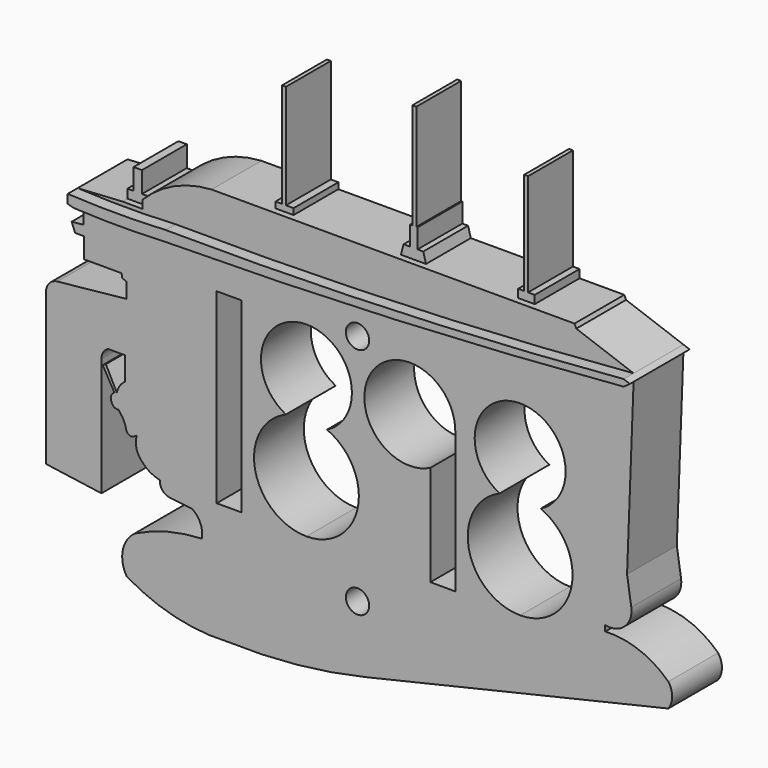
from build123d import *

# Parameters (mm, degrees)
F1_DEPTH = 12.7
F2_DEPTH = 12.7
F3_DEPTH = 15.24
F0_W     = 0.8031209019
F0_H     = 20.8792375506
F0_H_2   = 21.3003987877
F0_H_3   = 21.5899625402
F4_DEPTH = 11.43
F6_W     = 5.08
F6_H     = 38.1
F6_R     = 4.1999289977
F7_DEPTH = 25.4
F9_DEPTH = 25.4


# Not quite as in the source:
# - a feature names something its author has since deleted; it is built from what else it names


with BuildPart() as f1:
    # F0 (on Front) → F1 (new body)
    with BuildSketch(Plane.XZ):
        with BuildLine():
            Line((-48.7551556499, 16.502033492), (-48.7551556499, 13.4174126565))
            Line((-48.7551556499, 13.4174126565), (-62.8553717881, 11.9587710013))
            ThreePointArc((-62.8553717881, 11.9587710013), (-64.4593193904, 11.1699658138), (-65.1648855989, 9.527699739))
            Line((-65.1648855989, 9.527699739), (-65.1648855989, -21.5900078871))
            Line((-65.1648855989, -21.5900078871), (-53.8604057294, -23.1702051567))
            Line((-53.8604057294, -23.1702051567), (-53.8604057294, 1.0189516987))
            ThreePointArc((-53.8604057294, 1.0189516987), (-53.4996704115, 2.3010390091), (-52.5233172394, 3.2069155593))
            Line((-52.5233172394, 3.2069155593), (-49.036793639, 3.2069155593))
            Line((-49.036793639, 3.2069155593), (-49.036793639, -1.5386344666))
            ThreePointArc((-49.036793639, -1.5386344666), (-47.615617645, -3.4104534246), (-47.3704157715, -5.7478287601))
            Line((-47.3704157715, -5.7478287601), (-46.9190361118, -6.2988243644))
            ThreePointArc((-46.9190361118, -6.2988243644), (-46.2448724821, -6.7832935586), (-45.6504018941, -7.3627861985))
            ThreePointArc((-45.6504018941, -7.3627861985), (-45.2851101067, -8.4586657322), (-45.6504018941, -9.5545452658))
            ThreePointArc((-45.6504018941, -9.5545452658), (-46.1279766102, -10.0258883196), (-46.6583830297, -10.4368760494))
            ThreePointArc((-46.6583830297, -10.4368760494), (-46.8361198696, -11.8225114542), (-46.60965919, -13.2010220344))
            ThreePointArc((-46.60965919, -13.2010220344), (-44.7140636791, -15.6159662106), (-41.9303173119, -16.9105680327))
            ThreePointArc((-41.9303173119, -16.9105680327), (-41.4025572934, -18.5951701498), (-39.849619977, -19.4346941943))
            Line((-39.849619977, -19.4346941943), (-35.3891622198, -19.9264425199))
            ThreePointArc((-35.3891622198, -19.9264425199), (-25.5608590414, -18.8572797934), (-15.7824102789, -17.4010545015))
            ThreePointArc((-15.7824102789, -17.4010545015), (-8.2182486661, -13.3883283665), (-5.1937012606, -5.3776714064))
            Line((-5.1937012606, -5.3776714064), (38.9031486872, 1.6952896796))
            Line((38.9031486872, 1.6952896796), (48.6844740711, 1.6952896796))
            Line((48.6844740711, 1.6952896796), (48.9549487829, -13.394898735))
            ThreePointArc((48.9549487829, -13.394898735), (52.9202633868, -12.3483898503), (54.2744512358, -8.4773336607))
            Line((54.2744512358, -8.4773336607), (53.4126908814, -2.8367075716))
            Line((53.4126908814, -2.8367075716), (54.7520132328, 32.3448944531))
            ThreePointArc((54.7520132328, 32.3448944531), (8.06619556, 29.2264265692), (-38.7060455978, 27.9427323651))
            ThreePointArc((-38.7060455978, 27.9427323651), (-48.0915364769, 27.7060167093), (-57.477027356, 27.9427323651))
            Line((-57.477027356, 27.9427323651), (-57.477027356, 23.904802117))
            Line((-57.477027356, 23.904802117), (-59.946908801, 23.649297384))
            Line((-59.946908801, 23.649297384), (-59.2430122304, 21.8624826357))
            Line((-59.2430122304, 21.8624826357), (-57.4561974821, 21.8624826357))
            Line((-57.4561974821, 21.8624826357), (-57.4561974821, 17.7166229842))
            Line((-57.4561974821, 17.7166229842), (-49.7400154939, 17.7166229842))
            Line((-49.7400154939, 17.7166229842), (-49.6591787643, 16.9352005181))
            Line((-49.6591787643, 16.9352005181), (-48.7551556499, 16.502033492))
        make_face()
        with BuildLine():
            ThreePointArc((-47.3704157715, -5.7478287601), (-47.615617645, -3.4104534246), (-49.036793639, -1.5386344666))
            ThreePointArc((-49.036793639, -1.5386344666), (-50.1207303597, -2.6383216139), (-50.7394958839, -4.0530158787))
            ThreePointArc((-50.7394958839, -4.0530158787), (-49.7106058857, -4.489200491), (-49.2601067453, -5.5119038542))
            ThreePointArc((-49.2601067453, -5.5119038542), (-48.3211852646, -5.6888381711), (-47.4264473374, -6.0239849165))
            ThreePointArc((-47.4264473374, -6.0239849165), (-47.3962036519, -5.8863588755), (-47.3704157715, -5.7478287601))
        make_face()
        with BuildLine():
            ThreePointArc((-49.2601067453, -5.5119038542), (-49.7106058857, -4.489200491), (-50.7394958839, -4.0530158787))
            ThreePointArc((-50.7394958839, -4.0530158787), (-50.8140907016, -5.5738489648), (-50.3470855905, -7.0231259877))
            ThreePointArc((-50.3470855905, -7.0231259877), (-49.5443514855, -6.4539822041), (-49.2601067453, -5.5119038542))
        make_face()
        with BuildLine():
            ThreePointArc((-50.3470855905, -7.0231259877), (-50.8140907016, -5.5738489648), (-50.7394958839, -4.0530158787))
            ThreePointArc((-50.7394958839, -4.0530158787), (-50.9812103214, -4.1166962613), (-51.2089185655, -4.2197982303))
            ThreePointArc((-51.2089185655, -4.2197982303), (-51.743532248, -4.7258542326), (-51.9714604077, -5.4258208183))
            ThreePointArc((-51.9714604077, -5.4258208183), (-51.7264168334, -6.2602547319), (-51.186346321, -6.9419072469))
            ThreePointArc((-51.186346321, -6.9419072469), (-50.7704583506, -7.0211880502), (-50.3470855905, -7.0231259877))
        make_face()
        with BuildLine():
            ThreePointArc((-51.2089185655, -4.2197982303), (-50.9812103214, -4.1166962613), (-50.7394958839, -4.0530158787))
            Line((-50.7394958839, -4.0530158787), (-52.958683025, 0.3205834158))
            Line((-52.958683025, 0.3205834158), (-53.6059290171, -0.051631916))
            Line((-53.6059290171, -0.051631916), (-51.2089185655, -4.2197982303))
        make_face()
        with BuildLine():
            Line((-46.9190361118, -6.2988243644), (-47.3704157715, -5.7478287601))
            ThreePointArc((-47.3704157715, -5.7478287601), (-47.3962036519, -5.8863588755), (-47.4264473374, -6.0239849165))
            ThreePointArc((-47.4264473374, -6.0239849165), (-47.1691719509, -6.15481409), (-46.9190361118, -6.2988243644))
        make_face()
        with BuildLine():
            ThreePointArc((-49.5964513737, -8.0300319781), (-49.946242615, -7.507549809), (-50.3470855905, -7.0231259877))
            ThreePointArc((-50.3470855905, -7.0231259877), (-50.0092212706, -7.5544995086), (-49.5964513737, -8.0300319781))
        make_face()
        with BuildLine():
            ThreePointArc((-49.2601067453, -5.5119038542), (-49.5443514855, -6.4539822041), (-50.3470855905, -7.0231259877))
            ThreePointArc((-50.3470855905, -7.0231259877), (-49.946242615, -7.507549809), (-49.5964513737, -8.0300319781))
            ThreePointArc((-49.5964513737, -8.0300319781), (-49.3266753815, -8.2757089525), (-49.036793639, -8.4973050651))
            ThreePointArc((-49.036793639, -8.4973050651), (-48.0163521737, -7.4008033663), (-47.4264473374, -6.0239849165))
            ThreePointArc((-47.4264473374, -6.0239849165), (-48.3211852646, -5.6888381711), (-49.2601067453, -5.5119038542))
        make_face()
        with BuildLine():
            ThreePointArc((-46.9190361118, -6.2988243644), (-47.1691719509, -6.15481409), (-47.4264473374, -6.0239849165))
            ThreePointArc((-47.4264473374, -6.0239849165), (-48.0163521737, -7.4008033663), (-49.036793639, -8.4973050651))
            ThreePointArc((-49.036793639, -8.4973050651), (-49.3266753815, -8.2757089525), (-49.5964513737, -8.0300319781))
            ThreePointArc((-49.5964513737, -8.0300319781), (-49.1268650573, -8.9954240946), (-48.8306023576, -10.0272776016))
            ThreePointArc((-48.8306023576, -10.0272776016), (-48.4443790706, -10.7265299049), (-47.6917445685, -10.9942303294))
            ThreePointArc((-47.6917445685, -10.9942303294), (-47.1604512125, -10.7426456251), (-46.6583830297, -10.4368760494))
            ThreePointArc((-46.6583830297, -10.4368760494), (-46.6347395299, -10.3551418199), (-46.60965919, -10.2738369867))
            ThreePointArc((-46.60965919, -10.2738369867), (-45.8234576817, -8.6803013071), (-46.356693987, -6.9852709782))
            Line((-46.356693987, -6.9852709782), (-46.9190361118, -6.2988243644))
        make_face()
        with BuildLine():
            ThreePointArc((-45.6504018941, -7.3627861985), (-46.2448724821, -6.7832935586), (-46.9190361118, -6.2988243644))
            Line((-46.9190361118, -6.2988243644), (-46.356693987, -6.9852709782))
            ThreePointArc((-46.356693987, -6.9852709782), (-45.8234576817, -8.6803013071), (-46.60965919, -10.2738369867))
            ThreePointArc((-46.60965919, -10.2738369867), (-46.6347395299, -10.3551418199), (-46.6583830297, -10.4368760494))
            ThreePointArc((-46.6583830297, -10.4368760494), (-46.1279766102, -10.0258883196), (-45.6504018941, -9.5545452658))
            ThreePointArc((-45.6504018941, -9.5545452658), (-45.2851101067, -8.4586657322), (-45.6504018941, -7.3627861985))
        make_face()
        Polygon((48.9549487829, -14.5681889131), (48.9549487829, -13.394898735), (48.6844740711, 1.6952896796), (0, -6.1135082506), (0, -33.2036390901), (6.9897733629, -31.6629558802), (6.9897733629, -12.1476817876), (44.0394468606, -6.2050600536), (44.0394468606, -23.5927309841), (48.9549487829, -22.5092579032), align=None)
        with BuildLine():
            ThreePointArc((61.8351144011, -19.3772837126), (55.8950908573, -15.6334310122), (48.9549487829, -14.5681889131))
            Line((48.9549487829, -14.5681889131), (48.9549487829, -22.5092579032))
            Line((48.9549487829, -22.5092579032), (44.0394468606, -23.5927309841))
            Line((44.0394468606, -23.5927309841), (6.9897733629, -31.6629558802))
            Line((6.9897733629, -31.6629558802), (0, -33.2036390901))
            ThreePointArc((0, -33.2036390901), (-13.9786608203, -35.5041994352), (-28.1235985458, -36.2892299891))
            ThreePointArc((-28.1235985458, -36.2892299891), (-36.968923327, -35.9627176522), (-45.3792661428, -33.2036390901))
            ThreePointArc((-45.3792661428, -33.2036390901), (-46.9884285215, -30.9374841749), (-47.0181743808, -28.1582798204))
            ThreePointArc((-47.0181743808, -28.1582798204), (-49.5076846975, -31.9569932635), (-48.7172485904, -36.4294753708))
            ThreePointArc((-48.7172485904, -36.4294753708), (-38.8219806126, -40.4819745273), (-28.1747894096, -41.4701026827))
            ThreePointArc((-28.1747894096, -41.4701026827), (-13.9958743449, -40.9971425936), (0, -38.6774820627))
            Line((0, -38.6774820627), (61.8351144011, -24.218985916))
            ThreePointArc((61.8351144011, -24.218985916), (62.6222056643, -21.7981348143), (61.8351144011, -19.3772837126))
        make_face()
        Polygon((0, -6.1135082506), (48.6844740711, 1.6952896796), (38.9031486872, 1.6952896796), (-5.1937012606, -5.3776714064), align=None)
        Polygon((0, -33.2036390901), (0, -6.1135082506), (-5.1937012606, -5.3776714064), (-5.1937012606, -31.4487681253), align=None)
        with BuildLine():
            ThreePointArc((-15.7824102789, -17.4010545015), (-25.5608590414, -18.8572797934), (-35.3891622198, -19.9264425199))
            ThreePointArc((-35.3891622198, -19.9264425199), (-33.6624013857, -21.9793164564), (-33.3946987915, -24.6484604575))
            Line((-33.3946987915, -24.6484604575), (-33.3946987915, -29.0951598436))
            Line((-33.3946987915, -29.0951598436), (-28.4458585083, -27.9946736991))
            Line((-28.4458585083, -27.9946736991), (-28.4458585083, -31.1493985355))
            Line((-28.4458585083, -31.1493985355), (-16.4138842374, -28.6549646407))
            Line((-16.4138842374, -28.6549646407), (-17.5877343863, -27.2610168904))
            Line((-17.5877343863, -27.2610168904), (-5.1937012606, -31.4487681253))
            Line((-5.1937012606, -31.4487681253), (-5.1937012606, -5.3776714064))
            ThreePointArc((-5.1937012606, -5.3776714064), (-8.2182486661, -13.3883283665), (-15.7824102789, -17.4010545015))
        make_face()
        Polygon((6.9897733629, -31.6629558802), (44.0394468606, -23.5927309841), (44.0394468606, -6.2050600536), (6.9897733629, -12.1476817876), align=None)
        with BuildLine():
            ThreePointArc((-28.1235985458, -36.2892299891), (-13.9786608203, -35.5041994352), (0, -33.2036390901))
            Line((0, -33.2036390901), (-5.1937012606, -31.4487681253))
            Line((-5.1937012606, -31.4487681253), (-17.5877343863, -27.2610168904))
            Line((-17.5877343863, -27.2610168904), (-16.4138842374, -28.6549646407))
            Line((-16.4138842374, -28.6549646407), (-28.4458585083, -31.1493985355))
            Line((-28.4458585083, -31.1493985355), (-28.4458585083, -27.9946736991))
            Line((-28.4458585083, -27.9946736991), (-33.3946987915, -29.0951598436))
            Line((-33.3946987915, -29.0951598436), (-33.3946987915, -24.6484604575))
            ThreePointArc((-33.3946987915, -24.6484604575), (-40.3900375793, -25.6907170392), (-47.0181743808, -28.1582798204))
            ThreePointArc((-47.0181743808, -28.1582798204), (-46.9884285215, -30.9374841749), (-45.3792661428, -33.2036390901))
            ThreePointArc((-45.3792661428, -33.2036390901), (-36.968923327, -35.9627176522), (-28.1235985458, -36.2892299891))
        make_face()
    extrude(amount=F1_DEPTH)



with BuildPart() as f1b:
    # F0 (on Front) → F1, piece 2 (new body)
    with BuildSketch(Plane.XZ):
        with BuildLine():
            Line((-49.5634950364, 30.6502017175), (-58.7173150909, 30.0915159325))
            ThreePointArc((-58.7173150909, 30.0915159325), (-48.7116803443, 29.8224606957), (-38.7060455978, 30.0915159325))
            ThreePointArc((-38.7060455978, 30.0915159325), (8.0657939775, 30.8005791155), (54.7520132328, 33.7168574792))
            Line((54.7520132328, 33.7168574792), (43.0524877201, 37.9363596424))
            Line((43.0524877201, 37.9363596424), (42.6878245507, 38.7264558278))
            Line((42.6878245507, 38.7264558278), (33.556767168, 38.7264558278))
            Line((33.556767168, 38.7264558278), (30.1818160021, 38.7264558278))
            Line((30.1818160021, 38.7264558278), (11.3595948708, 38.7264558278))
            Line((11.3595948708, 38.7264558278), (6.237627371, 38.7264558278))
            Line((6.237627371, 38.7264558278), (-15.6707727532, 38.7264558278))
            Line((-15.6707727532, 38.7264558278), (-19.3496172971, 38.7264558278))
            Line((-19.3496172971, 38.7264558278), (-31.3758637064, 38.7264558278))
            ThreePointArc((-31.3758637064, 38.7264558278), (-39.0221039671, 36.8382050442), (-45.4714367213, 32.3175205636))
            Line((-45.4714367213, 32.3175205636), (-45.4714367213, 30.6502017175))
            Line((-45.4714367213, 30.6502017175), (-49.5634950364, 30.6502017175))
        make_face()
    extrude(amount=F1_DEPTH)


with BuildPart() as f2:
    # F0 (on Front) → F2 (new body)
    with BuildSketch(Plane.XZ):
        with BuildLine():
            ThreePointArc((-46.9190361118, -6.2988243644), (-47.1691719509, -6.15481409), (-47.4264473374, -6.0239849165))
            ThreePointArc((-47.4264473374, -6.0239849165), (-48.0163521737, -7.4008033663), (-49.036793639, -8.4973050651))
            ThreePointArc((-49.036793639, -8.4973050651), (-49.3266753815, -8.2757089525), (-49.5964513737, -8.0300319781))
            ThreePointArc((-49.5964513737, -8.0300319781), (-49.1268650573, -8.9954240946), (-48.8306023576, -10.0272776016))
            ThreePointArc((-48.8306023576, -10.0272776016), (-48.4443790706, -10.7265299049), (-47.6917445685, -10.9942303294))
            ThreePointArc((-47.6917445685, -10.9942303294), (-47.1604512125, -10.7426456251), (-46.6583830297, -10.4368760494))
            ThreePointArc((-46.6583830297, -10.4368760494), (-46.6347395299, -10.3551418199), (-46.60965919, -10.2738369867))
            ThreePointArc((-46.60965919, -10.2738369867), (-45.8234576817, -8.6803013071), (-46.356693987, -6.9852709782))
            Line((-46.356693987, -6.9852709782), (-46.9190361118, -6.2988243644))
        make_face()
        with BuildLine():
            ThreePointArc((-49.2601067453, -5.5119038542), (-49.5443514855, -6.4539822041), (-50.3470855905, -7.0231259877))
            ThreePointArc((-50.3470855905, -7.0231259877), (-49.946242615, -7.507549809), (-49.5964513737, -8.0300319781))
            ThreePointArc((-49.5964513737, -8.0300319781), (-49.3266753815, -8.2757089525), (-49.036793639, -8.4973050651))
            ThreePointArc((-49.036793639, -8.4973050651), (-48.0163521737, -7.4008033663), (-47.4264473374, -6.0239849165))
            ThreePointArc((-47.4264473374, -6.0239849165), (-48.3211852646, -5.6888381711), (-49.2601067453, -5.5119038542))
        make_face()
        with BuildLine():
            ThreePointArc((-45.6504018941, -7.3627861985), (-46.2448724821, -6.7832935586), (-46.9190361118, -6.2988243644))
            Line((-46.9190361118, -6.2988243644), (-46.356693987, -6.9852709782))
            ThreePointArc((-46.356693987, -6.9852709782), (-45.8234576817, -8.6803013071), (-46.60965919, -10.2738369867))
            ThreePointArc((-46.60965919, -10.2738369867), (-46.6347395299, -10.3551418199), (-46.6583830297, -10.4368760494))
            ThreePointArc((-46.6583830297, -10.4368760494), (-46.1279766102, -10.0258883196), (-45.6504018941, -9.5545452658))
            ThreePointArc((-45.6504018941, -9.5545452658), (-45.2851101067, -8.4586657322), (-45.6504018941, -7.3627861985))
        make_face()
        with BuildLine():
            Line((-46.9190361118, -6.2988243644), (-47.3704157715, -5.7478287601))
            ThreePointArc((-47.3704157715, -5.7478287601), (-47.3962036519, -5.8863588755), (-47.4264473374, -6.0239849165))
            ThreePointArc((-47.4264473374, -6.0239849165), (-47.1691719509, -6.15481409), (-46.9190361118, -6.2988243644))
        make_face()
        with BuildLine():
            ThreePointArc((-49.2601067453, -5.5119038542), (-49.7106058857, -4.489200491), (-50.7394958839, -4.0530158787))
            ThreePointArc((-50.7394958839, -4.0530158787), (-50.8140907016, -5.5738489648), (-50.3470855905, -7.0231259877))
            ThreePointArc((-50.3470855905, -7.0231259877), (-49.5443514855, -6.4539822041), (-49.2601067453, -5.5119038542))
        make_face()
    extrude(amount=F2_DEPTH)


with BuildPart() as f1_1:
    add(f1.part)

    add(f1b.part)  # F3 merges F1b
    # F0 (on Front) → F3 (join)
    with BuildSketch(Plane.XZ):
        with BuildLine():
            Line((-58.7173150909, 28.2865388137), (-57.477027356, 27.9427323651))
            ThreePointArc((-57.477027356, 27.9427323651), (-48.0915364769, 27.7060167093), (-38.7060455978, 27.9427323651))
            ThreePointArc((-38.7060455978, 27.9427323651), (8.06619556, 29.2264265692), (54.7520132328, 32.3448944531))
            Line((54.7520132328, 32.3448944531), (56.0283269774, 33.2565474777))
            Line((56.0283269774, 33.2565474777), (54.7520132328, 33.7168574792))
            ThreePointArc((54.7520132328, 33.7168574792), (8.0657939775, 30.8005791155), (-38.7060455978, 30.0915159325))
            ThreePointArc((-38.7060455978, 30.0915159325), (-48.7116803443, 29.8224606957), (-58.7173150909, 30.0915159325))
            Line((-58.7173150909, 30.0915159325), (-58.7173150909, 28.2865388137))
        make_face()
    extrude(amount=F3_DEPTH)

    # F0 (on Front) → F4 (join)
    with BuildSketch(Plane.XZ):
        Polygon((-49.5634950364, 32.4551788364), (-49.5634950364, 30.6502017175), (-45.4714367213, 30.6502017175), (-45.4714367213, 32.3175205636), (-45.4714367213, 32.4551788364), (-46.6116432115, 32.4551788364), (-46.6116432115, 36.7413145776), (-48.3172012532, 36.7413145776), (-48.3172012532, 32.4551788364), align=None)
        Polygon((-19.3496172971, 39.9737632714), (-19.3496172971, 38.7264558278), (-15.6707727532, 38.7264558278), (-15.6707727532, 39.9737632714), (-17.2171857255, 39.9737632714), (-18.0203066274, 39.9737632714), align=None)
        Polygon((6.7892512256, 40.7851440797), (6.237627371, 38.7264558278), (11.3595948708, 38.7264558278), (10.8079710163, 40.7851440797), (9.6353090061, 40.7851440797), (9.6353090061, 44.7442179937), (9.3757620237, 44.7442179937), (8.5726411218, 44.7442179937), (8.1109651281, 44.7442179937), (8.1109651281, 40.7851440797), align=None)
        with Locations((31.7935269116, 50.8345432838)):
            Rectangle(F0_W, F0_H)
        Polygon((30.1818160021, 38.7264558278), (33.556767168, 38.7264558278), (33.556767168, 40.3949245085), (32.1950873626, 40.3949245085), (31.3919664607, 40.3949245085), (30.1818160021, 40.3949245085), align=None)
        with Locations((-17.6187461764, 50.6239626653)):
            Rectangle(F0_W, F0_H_2)
        with Locations((8.9742015728, 55.5391992638)):
            Rectangle(F0_W, F0_H_3)
    extrude(amount=F4_DEPTH)


with BuildPart() as f2_1:
    add(f2.part)

    # F5: union F1
    add(f1_1.part)

    # F6 (on face) → F7 (cut)
    with BuildSketch(Plane.XZ.offset(12.7)):
        with Locations((-27.8038021288, 1.7426949936)):
            Rectangle(F6_W, F6_H)
        with BuildLine():
            Line((-12.0248878375, 16.1970947476), (-12.0248878375, 20.7926949936))
            ThreePointArc((-12.0248878375, 20.7926949936), (-21.0509501852, 13.6685212457), (-16.2184503735, 3.2344137772))
            ThreePointArc((-16.2184503735, 3.2344137772), (-14.1649165015, 3.8743114334), (-12.0248878375, 4.0905235764))
            Line((-12.0248878375, 4.0905235764), (-12.0248878375, 6.8284372443))
            ThreePointArc((-12.0248878375, 6.8284372443), (-16.7092165891, 11.512765996), (-12.0248878375, 16.1970947476))
        make_face()
        with BuildLine():
            ThreePointArc((-2.7449588398, 11.512765996), (-5.4629871143, 18.0746667192), (-12.0248878375, 20.7926949936))
            Line((-12.0248878375, 20.7926949936), (-12.0248878375, 16.1970947476))
            ThreePointArc((-12.0248878375, 16.1970947476), (-8.7125672119, 14.8250866216), (-7.3405590858, 11.512765996))
            ThreePointArc((-7.3405590858, 11.512765996), (-8.7125672119, 8.2004453704), (-12.0248878375, 6.8284372443))
            Line((-12.0248878375, 6.8284372443), (-12.0248878375, 4.0905235764))
            ThreePointArc((-12.0248878375, 4.0905235764), (-9.8848591734, 3.8743114334), (-7.8313253015, 3.2344137772))
            ThreePointArc((-7.8313253015, 3.2344137772), (-4.1181487883, 6.6547252582), (-2.7449588398, 11.512765996))
        make_face()
        with BuildLine():
            ThreePointArc((-12.0248878375, 2.2328369983), (-9.8691325877, 2.4867036483), (-7.8313253015, 3.2344137772))
            ThreePointArc((-7.8313253015, 3.2344137772), (-9.8848591734, 3.8743114334), (-12.0248878375, 4.0905235764))
            Line((-12.0248878375, 4.0905235764), (-12.0248878375, 2.2328369983))
        make_face()
        with BuildLine():
            ThreePointArc((-12.0248878375, 4.0905235764), (-14.1649165015, 3.8743114334), (-16.2184503735, 3.2344137772))
            ThreePointArc((-16.2184503735, 3.2344137772), (-14.1806430872, 2.4867036483), (-12.0248878375, 2.2328369983))
            Line((-12.0248878375, 2.2328369983), (-12.0248878375, 4.0905235764))
        make_face()
        with BuildLine():
            ThreePointArc((-16.2184503735, 3.2344137772), (-22.5075899858, -8.748419379), (-12.0248878375, -17.3073050064))
            Line((-12.0248878375, -17.3073050064), (-12.0248878375, -12.3384351215))
            ThreePointArc((-12.0248878375, -12.3384351215), (-17.754932244, -6.608390715), (-12.0248878375, -0.8783463084))
            Line((-12.0248878375, -0.8783463084), (-12.0248878375, 2.2328369983))
            ThreePointArc((-12.0248878375, 2.2328369983), (-14.1806430872, 2.4867036483), (-16.2184503735, 3.2344137772))
        make_face()
        with BuildLine():
            Line((-12.0248878375, -12.3384351215), (-12.0248878375, -17.3073050064))
            ThreePointArc((-12.0248878375, -17.3073050064), (-4.4596129907, -14.1736655617), (-1.3259735461, -6.608390715))
            ThreePointArc((-1.3259735461, -6.608390715), (-3.0992692829, -0.709229721), (-7.8313253015, 3.2344137772))
            ThreePointArc((-7.8313253015, 3.2344137772), (-9.8691325877, 2.4867036483), (-12.0248878375, 2.2328369983))
            Line((-12.0248878375, 2.2328369983), (-12.0248878375, -0.8783463084))
            ThreePointArc((-12.0248878375, -0.8783463084), (-7.9731345811, -2.5566374586), (-6.2948434309, -6.608390715))
            ThreePointArc((-6.2948434309, -6.608390715), (-7.9731345811, -10.6601439714), (-12.0248878375, -12.3384351215))
        make_face()
        with BuildLine():
            ThreePointArc((18.3548991555, 11.512765996), (15.6368709195, 18.0746666807), (9.0749702668, 20.7926949936))
            ThreePointArc((9.0749702668, 20.7926949936), (0.0497375677, 9.3535395382), (13.2748991555, 3.2376419113))
            Line((13.2748991555, 3.2376419113), (13.2748991555, 11.512765996))
            Line((13.2748991555, 11.512765996), (18.3548991555, 11.512765996))
        make_face()
        with Locations((9.0749701579, 11.512765996)):
            Circle(F6_R, mode=Mode.SUBTRACT)
        with BuildLine():
            ThreePointArc((13.2748991555, 3.2376419113), (16.983577023, 6.6577665465), (18.3548991555, 11.512765996))
            Line((18.3548991555, 11.512765996), (13.2748991555, 11.512765996))
            Line((13.2748991555, 11.512765996), (13.2748991555, 3.2376419113))
        make_face()
        with BuildLine():
            Line((13.2748991555, 3.2376419113), (13.2748991555, -17.3073050064))
            Line((13.2748991555, -17.3073050064), (18.3548991555, -17.3073050064))
            Line((18.3548991555, -17.3073050064), (18.3548991555, 11.512765996))
            ThreePointArc((18.3548991555, 11.512765996), (16.983577023, 6.6577665465), (13.2748991555, 3.2376419113))
        make_face()
        with BuildLine():
            Line((31.5938134469, 16.5285051951), (31.5938134469, 20.7926949936))
            ThreePointArc((31.5938134469, 20.7926949936), (22.5677510992, 13.6685212457), (27.4002509109, 3.2344137772))
            ThreePointArc((27.4002509109, 3.2344137772), (29.4537847829, 3.8743114334), (31.5938134469, 4.0905235764))
            Line((31.5938134469, 4.0905235764), (31.5938134469, 6.4970267968))
            ThreePointArc((31.5938134469, 6.4970267968), (26.5780742478, 11.512765996), (31.5938134469, 16.5285051951))
        make_face()
        with BuildLine():
            ThreePointArc((40.8737424446, 11.512765996), (38.1557141701, 18.0746667192), (31.5938134469, 20.7926949936))
            Line((31.5938134469, 20.7926949936), (31.5938134469, 16.5285051951))
            ThreePointArc((31.5938134469, 16.5285051951), (35.1404766473, 15.0594291964), (36.609552646, 11.512765996))
            ThreePointArc((36.609552646, 11.512765996), (35.1404766473, 7.9661027956), (31.5938134469, 6.4970267968))
            Line((31.5938134469, 6.4970267968), (31.5938134469, 4.0905235764))
            ThreePointArc((31.5938134469, 4.0905235764), (33.7338421109, 3.8743114334), (35.7873759829, 3.2344137772))
            ThreePointArc((35.7873759829, 3.2344137772), (39.5005524961, 6.6547252582), (40.8737424446, 11.512765996))
        make_face()
        with BuildLine():
            ThreePointArc((31.5938134469, 2.2328369983), (33.7495686967, 2.4867036483), (35.7873759829, 3.2344137772))
            ThreePointArc((35.7873759829, 3.2344137772), (33.7338421109, 3.8743114334), (31.5938134469, 4.0905235764))
            Line((31.5938134469, 4.0905235764), (31.5938134469, 2.2328369983))
        make_face()
        with BuildLine():
            ThreePointArc((31.5938134469, 4.0905235764), (29.4537847829, 3.8743114334), (27.4002509109, 3.2344137772))
            ThreePointArc((27.4002509109, 3.2344137772), (29.4380581972, 2.4867036483), (31.5938134469, 2.2328369983))
            Line((31.5938134469, 2.2328369983), (31.5938134469, 4.0905235764))
        make_face()
        with BuildLine():
            ThreePointArc((31.5938134469, 2.2328369983), (29.4380581972, 2.4867036483), (27.4002509109, 3.2344137772))
            ThreePointArc((27.4002509109, 3.2344137772), (21.1111112985, -8.748419379), (31.5938134469, -17.3073050064))
            Line((31.5938134469, -17.3073050064), (31.5938134469, -12.4269906531))
            ThreePointArc((31.5938134469, -12.4269906531), (25.7752135088, -6.608390715), (31.5938134469, -0.7897907769))
            Line((31.5938134469, -0.7897907769), (31.5938134469, 2.2328369983))
        make_face()
        with BuildLine():
            Line((31.5938134469, -12.4269906531), (31.5938134469, -17.3073050064))
            ThreePointArc((31.5938134469, -17.3073050064), (39.1590882937, -14.1736655617), (42.2927277383, -6.608390715))
            ThreePointArc((42.2927277383, -6.608390715), (40.5194320014, -0.709229721), (35.7873759829, 3.2344137772))
            ThreePointArc((35.7873759829, 3.2344137772), (33.7495686967, 2.4867036483), (31.5938134469, 2.2328369983))
            Line((31.5938134469, 2.2328369983), (31.5938134469, -0.7897907769))
            ThreePointArc((31.5938134469, -0.7897907769), (35.7081849202, -2.4940192417), (37.412413385, -6.608390715))
            ThreePointArc((37.412413385, -6.608390715), (35.7081849202, -10.7227621882), (31.5938134469, -12.4269906531))
        make_face()
        with BuildLine():
            Line((-12.0248878375, 11.512765996), (-12.0248878375, 16.1970947476))
            ThreePointArc((-12.0248878375, 16.1970947476), (-16.7092165891, 11.512765996), (-12.0248878375, 6.8284372443))
            Line((-12.0248878375, 6.8284372443), (-12.0248878375, 11.512765996))
        make_face()
        with BuildLine():
            ThreePointArc((-7.3405590858, 11.512765996), (-8.7125672119, 14.8250866216), (-12.0248878375, 16.1970947476))
            Line((-12.0248878375, 16.1970947476), (-12.0248878375, 11.512765996))
            Line((-12.0248878375, 11.512765996), (-12.0248878375, 6.8284372443))
            ThreePointArc((-12.0248878375, 6.8284372443), (-8.7125672119, 8.2004453704), (-7.3405590858, 11.512765996))
        make_face()
        with BuildLine():
            Line((-12.0248878375, -0.8783463084), (-12.0248878375, -12.3384351215))
            ThreePointArc((-12.0248878375, -12.3384351215), (-7.9731345811, -10.6601439714), (-6.2948434309, -6.608390715))
            ThreePointArc((-6.2948434309, -6.608390715), (-7.9731345811, -2.5566374586), (-12.0248878375, -0.8783463084))
        make_face()
        with BuildLine():
            ThreePointArc((-12.0248878375, -0.8783463084), (-17.754932244, -6.608390715), (-12.0248878375, -12.3384351215))
            Line((-12.0248878375, -12.3384351215), (-12.0248878375, -0.8783463084))
        make_face()
        with Locations((9.0749701579, 11.512765996)):
            Circle(F6_R)
        with BuildLine():
            ThreePointArc((36.609552646, 11.512765996), (35.1404766473, 15.0594291964), (31.5938134469, 16.5285051951))
            Line((31.5938134469, 16.5285051951), (31.5938134469, 6.4970267968))
            ThreePointArc((31.5938134469, 6.4970267968), (35.1404766473, 7.9661027956), (36.609552646, 11.512765996))
        make_face()
        with BuildLine():
            Line((31.5938134469, 6.4970267968), (31.5938134469, 16.5285051951))
            ThreePointArc((31.5938134469, 16.5285051951), (26.5780742478, 11.512765996), (31.5938134469, 6.4970267968))
        make_face()
        with BuildLine():
            Line((31.5938134469, -0.7897907769), (31.5938134469, -12.4269906531))
            ThreePointArc((31.5938134469, -12.4269906531), (35.7081849202, -10.7227621882), (37.412413385, -6.608390715))
            ThreePointArc((37.412413385, -6.608390715), (35.7081849202, -2.4940192417), (31.5938134469, -0.7897907769))
        make_face()
        with BuildLine():
            ThreePointArc((31.5938134469, -0.7897907769), (25.7752135088, -6.608390715), (31.5938134469, -12.4269906531))
            Line((31.5938134469, -12.4269906531), (31.5938134469, -0.7897907769))
        make_face()
    extrude(amount=-F7_DEPTH, mode=Mode.SUBTRACT)

    # F8 (on face) → F9 (cut)
    with BuildSketch(Plane.XZ.offset(12.7)):
        with BuildLine():
            ThreePointArc((0.7787104972, 22.0298973173), (-3.2863375255, 23.71369534), (-1.6025395028, 19.6486473173))
            ThreePointArc((-1.6025395028, 19.6486473173), (0.0812585199, 20.3460992946), (0.7787104972, 22.0298973173))
        make_face()
        with BuildLine():
            ThreePointArc((0.7787104972, -25.5951026827), (0.0812585199, -23.91130466), (-1.6025395028, -23.2138526827))
            ThreePointArc((-1.6025395028, -23.2138526827), (-3.2863375255, -27.2789007054), (0.7787104972, -25.5951026827))
        make_face()
    extrude(amount=-F9_DEPTH, mode=Mode.SUBTRACT)


solid = f2_1.part
